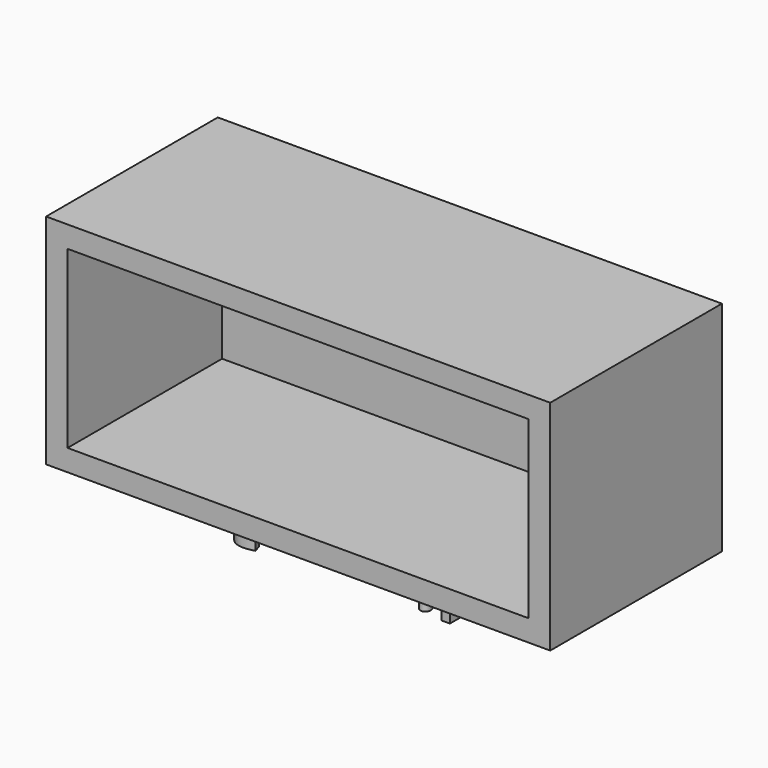
from build123d import *

# Parameters (mm, degrees)
F0_W         = 59.6595518291
F0_H         = 25.8226264268
F1_DEPTH     = 25.4
F2_T         = -2.54
F3_TEXT_SIZE = 12.408499606
F4_DEPTH     = 5.08


# Not quite as in the source:
# - Text() gives the source's letters only with a copy of the font that has no kerning and outlines rounded to 1/6400 em; it was checked with that copy


with BuildPart() as f1:
    # F0 (on Front) → F1 (new body)
    with BuildSketch(Plane.XZ):
        with Locations((29.8297759145, -12.9113132134)):
            Rectangle(F0_W, F0_H)
    extrude(amount=F1_DEPTH)

    # F2
    f2_openings = [f1.faces().sort_by_distance(p)[0] for p in [
        (29.829776, -25.4, -12.911313),
    ]]
    offset(amount=F2_T, openings=f2_openings)

    # F3 (on face) → F4 (join)
    with BuildSketch(Plane(origin=(0, 0, -25.8226264268), x_dir=(1, 0, 0), z_dir=(0, 0, -1))):
        with Locations((15.088734217, 9.9204964936)):
            Text('family', F3_TEXT_SIZE, font='Open Sans', text_align=(TextAlign.LEFT, TextAlign.BOTTOM))
    extrude(amount=F4_DEPTH)


solid = f1.part
